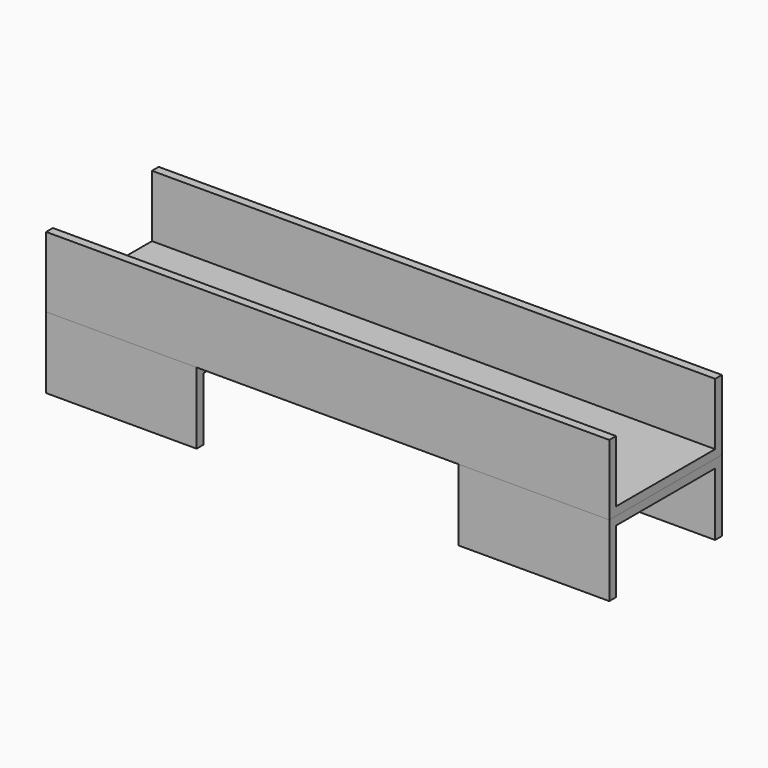
from build123d import *

# Parameters (mm, degrees)
F0_W     = 200
F0_H     = 25
F1_DEPTH = 50
F2_W     = 44
F2_H     = 22
F3_DEPTH = 200.001
F4_W     = 53.4567855299
F4_H     = 50
F5_DEPTH = 25.4
F6_W     = 44
F6_H     = 22.4
F7_DEPTH = 200.001


# Not quite as in the source:
# - a feature names something its author has since deleted; it is built from what else it names


with BuildPart() as f1:
    # F0 (on Front) → F1 (new body)
    with BuildSketch(Plane.XZ):
        Rectangle(F0_W, F0_H)
    extrude(amount=F1_DEPTH)

    # F2 (on face) → F3 (cut, through all)
    with BuildSketch(Plane.YZ.offset(100)):
        with Locations((-25, 1.5)):
            Rectangle(F2_W, F2_H)
    extrude(amount=-F3_DEPTH, mode=Mode.SUBTRACT)


with BuildPart() as f5:
    # F4 (on face) → F5 (new body)
    with BuildSketch(Plane(origin=(0, 0, -12.5), x_dir=(1, 0, 0), z_dir=(0, 0, -1))):
        with Locations((-73.2716072351, 25)):
            Rectangle(F4_W, F4_H)
    extrude(amount=F5_DEPTH)

    # F6 (on face) → F7 (cut, through all)
    with BuildSketch(Plane(origin=(-100, 0, 0), x_dir=(0, -1, 0), z_dir=(-1, 0, 0))):
        with Locations((25, -26.7)):
            Rectangle(F6_W, F6_H)
    extrude(amount=-F7_DEPTH, mode=Mode.SUBTRACT)


with BuildPart() as f8_1:
    # F8: instance of F5
    add(f5.part.mirror(Plane.YZ))


solid = Compound([f1.part, f5.part, f8_1.part])
